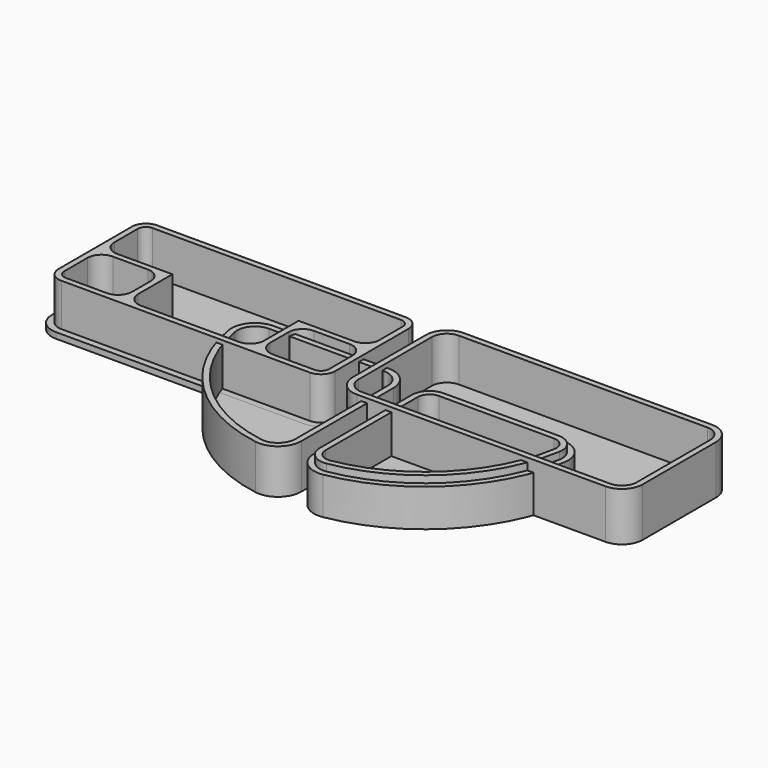
from build123d import *

# Parameters (mm, degrees)
F2_DEPTH = 3.175
F3_DEPTH = 24.13
F4_DEPTH = 20.32
F5_DEPTH = 24.13
F6_DEPTH = 3.175
F7_DEPTH = 26.275
F8_DEPTH = 26.5
F9_DEPTH = 3.175


# Not quite as in the source:
# - a feature names something its author has since deleted; it is built from what else it names


with BuildPart() as f2:
    # F1 (on Top) → F2 (new body)
    with BuildSketch(Plane.XY):
        with BuildLine():
            ThreePointArc((44.45, 31.75), (40.7302561211, 40.7302561211), (31.75, 44.45))
            Line((31.75, 44.45), (-30.6842132454, 44.45))
            ThreePointArc((-30.6842132454, 44.45), (-40.3839984664, 39.9478147495), (-43.2065821196, 29.6333333333))
            ThreePointArc((-43.2065821196, 29.6333333333), (-18.4117928475, -18.4117928475), (29.6333333333, -43.2065821196))
            ThreePointArc((29.6333333333, -43.2065821196), (39.9478147495, -40.3839984664), (44.45, -30.6842132454))
            Line((44.45, -30.6842132454), (44.45, 31.75))
        make_face()
        with BuildLine():
            ThreePointArc((31.75, 41.275), (38.4851920908, 38.4851920908), (41.275, 31.75))
            Line((41.275, 31.75), (41.275, -30.6842132454))
            ThreePointArc((41.275, -30.6842132454), (37.8983610621, -37.9590521611), (30.1625, -40.075989901))
            ThreePointArc((30.1625, -40.075989901), (-16.1667288172, -16.1667288172), (-40.075989901, 30.1625))
            ThreePointArc((-40.075989901, 30.1625), (-37.9590521611, 37.8983610621), (-30.6842132454, 41.275))
            Line((-30.6842132454, 41.275), (31.75, 41.275))
        make_face(mode=Mode.SUBTRACT)
        with BuildLine():
            Line((41.275, -30.6842132454), (41.275, 31.75))
            ThreePointArc((41.275, 31.75), (38.4851920908, 38.4851920908), (31.75, 41.275))
            Line((31.75, 41.275), (-30.6842132454, 41.275))
            ThreePointArc((-30.6842132454, 41.275), (-37.9590521611, 37.8983610621), (-40.075989901, 30.1625))
            ThreePointArc((-40.075989901, 30.1625), (-16.1667288172, -16.1667288172), (30.1625, -40.075989901))
            ThreePointArc((30.1625, -40.075989901), (37.8983610621, -37.9590521611), (41.275, -30.6842132454))
        make_face()
        with BuildLine():
            Line((-30.6842132454, 38.1), (31.75, 38.1))
            ThreePointArc((31.75, 38.1), (36.2401280605, 36.2401280605), (38.1, 31.75))
            Line((38.1, 31.75), (38.1, -30.6842132454))
            ThreePointArc((38.1, -30.6842132454), (35.8489073747, -35.5341058559), (30.6916666667, -36.9453976825))
            ThreePointArc((30.6916666667, -36.9453976825), (-13.9216647869, -13.9216647869), (-36.9453976825, 30.6916666667))
            ThreePointArc((-36.9453976825, 30.6916666667), (-35.5341058559, 35.8489073747), (-30.6842132454, 38.1))
        make_face(mode=Mode.SUBTRACT)
        with BuildLine():
            ThreePointArc((38.1, 31.75), (36.2401280605, 36.2401280605), (31.75, 38.1))
            Line((31.75, 38.1), (-30.6842132454, 38.1))
            ThreePointArc((-30.6842132454, 38.1), (-35.5341058559, 35.8489073747), (-36.9453976825, 30.6916666667))
            ThreePointArc((-36.9453976825, 30.6916666667), (-13.9216647869, -13.9216647869), (30.6916666667, -36.9453976825))
            ThreePointArc((30.6916666667, -36.9453976825), (35.8489073747, -35.5341058559), (38.1, -30.6842132454))
            Line((38.1, -30.6842132454), (38.1, 31.75))
        make_face()
    extrude(amount=F2_DEPTH)

    # F1 (on Top) → F3 (join)
    with BuildSketch(Plane.XY):
        with BuildLine():
            ThreePointArc((44.45, 31.75), (40.7302561211, 40.7302561211), (31.75, 44.45))
            Line((31.75, 44.45), (-30.6842132454, 44.45))
            ThreePointArc((-30.6842132454, 44.45), (-40.3839984664, 39.9478147495), (-43.2065821196, 29.6333333333))
            ThreePointArc((-43.2065821196, 29.6333333333), (-18.4117928475, -18.4117928475), (29.6333333333, -43.2065821196))
            ThreePointArc((29.6333333333, -43.2065821196), (39.9478147495, -40.3839984664), (44.45, -30.6842132454))
            Line((44.45, -30.6842132454), (44.45, 31.75))
        make_face()
        with BuildLine():
            ThreePointArc((31.75, 41.275), (38.4851920908, 38.4851920908), (41.275, 31.75))
            Line((41.275, 31.75), (41.275, -30.6842132454))
            ThreePointArc((41.275, -30.6842132454), (37.8983610621, -37.9590521611), (30.1625, -40.075989901))
            ThreePointArc((30.1625, -40.075989901), (-16.1667288172, -16.1667288172), (-40.075989901, 30.1625))
            ThreePointArc((-40.075989901, 30.1625), (-37.9590521611, 37.8983610621), (-30.6842132454, 41.275))
            Line((-30.6842132454, 41.275), (31.75, 41.275))
        make_face(mode=Mode.SUBTRACT)
    extrude(amount=F3_DEPTH)


with BuildPart() as f2b:
    # F1 (on Top) → F2, piece 2 (new body)
    with BuildSketch(Plane.XY):
        with BuildLine():
            Line((51.308, 31.75), (51.308, -30.6842132454))
            ThreePointArc((51.308, -30.6842132454), (55.8101852505, -40.3839984664), (66.1246666667, -43.2065821196))
            ThreePointArc((66.1246666667, -43.2065821196), (114.1697928475, -18.4117928475), (138.9645821196, 29.6333333333))
            ThreePointArc((138.9645821196, 29.6333333333), (136.1419984664, 39.9478147495), (126.4422132454, 44.45))
            Line((126.4422132454, 44.45), (64.008, 44.45))
            ThreePointArc((64.008, 44.45), (55.0277438789, 40.7302561211), (51.308, 31.75))
        make_face()
        with BuildLine():
            ThreePointArc((65.5955, -40.075989901), (57.8596389379, -37.9590521611), (54.483, -30.6842132454))
            Line((54.483, -30.6842132454), (54.483, 31.75))
            ThreePointArc((54.483, 31.75), (57.2728079092, 38.4851920908), (64.008, 41.275))
            Line((64.008, 41.275), (126.4422132454, 41.275))
            ThreePointArc((126.4422132454, 41.275), (133.7170521611, 37.8983610621), (135.833989901, 30.1625))
            ThreePointArc((135.833989901, 30.1625), (111.9247288172, -16.1667288172), (65.5955, -40.075989901))
        make_face(mode=Mode.SUBTRACT)
        with BuildLine():
            Line((54.483, 31.75), (54.483, -30.6842132454))
            ThreePointArc((54.483, -30.6842132454), (57.8596389379, -37.9590521611), (65.5955, -40.075989901))
            ThreePointArc((65.5955, -40.075989901), (111.9247288172, -16.1667288172), (135.833989901, 30.1625))
            ThreePointArc((135.833989901, 30.1625), (133.7170521611, 37.8983610621), (126.4422132454, 41.275))
            Line((126.4422132454, 41.275), (64.008, 41.275))
            ThreePointArc((64.008, 41.275), (57.2728079092, 38.4851920908), (54.483, 31.75))
        make_face()
        with BuildLine():
            ThreePointArc((65.0663333333, -36.9453976825), (59.9090926253, -35.5341058559), (57.658, -30.6842132454))
            Line((57.658, -30.6842132454), (57.658, 31.75))
            ThreePointArc((57.658, 31.75), (59.5178719395, 36.2401280605), (64.008, 38.1))
            Line((64.008, 38.1), (126.4422132454, 38.1))
            ThreePointArc((126.4422132454, 38.1), (131.2921058559, 35.8489073747), (132.7033976825, 30.6916666667))
            ThreePointArc((132.7033976825, 30.6916666667), (109.6796647869, -13.9216647869), (65.0663333333, -36.9453976825))
        make_face(mode=Mode.SUBTRACT)
        with BuildLine():
            Line((57.658, 31.75), (57.658, -30.6842132454))
            ThreePointArc((57.658, -30.6842132454), (59.9090926253, -35.5341058559), (65.0663333333, -36.9453976825))
            ThreePointArc((65.0663333333, -36.9453976825), (109.6796647869, -13.9216647869), (132.7033976825, 30.6916666667))
            ThreePointArc((132.7033976825, 30.6916666667), (131.2921058559, 35.8489073747), (126.4422132454, 38.1))
            Line((126.4422132454, 38.1), (64.008, 38.1))
            ThreePointArc((64.008, 38.1), (59.5178719395, 36.2401280605), (57.658, 31.75))
        make_face()
    extrude(amount=F2_DEPTH)

    # F1 (on Top) → F4 (join)
    with BuildSketch(Plane.XY):
        with BuildLine():
            Line((51.308, 31.75), (51.308, -30.6842132454))
            ThreePointArc((51.308, -30.6842132454), (55.8101852505, -40.3839984664), (66.1246666667, -43.2065821196))
            ThreePointArc((66.1246666667, -43.2065821196), (114.1697928475, -18.4117928475), (138.9645821196, 29.6333333333))
            ThreePointArc((138.9645821196, 29.6333333333), (136.1419984664, 39.9478147495), (126.4422132454, 44.45))
            Line((126.4422132454, 44.45), (64.008, 44.45))
            ThreePointArc((64.008, 44.45), (55.0277438789, 40.7302561211), (51.308, 31.75))
        make_face()
        with BuildLine():
            ThreePointArc((65.5955, -40.075989901), (57.8596389379, -37.9590521611), (54.483, -30.6842132454))
            Line((54.483, -30.6842132454), (54.483, 31.75))
            ThreePointArc((54.483, 31.75), (57.2728079092, 38.4851920908), (64.008, 41.275))
            Line((64.008, 41.275), (126.4422132454, 41.275))
            ThreePointArc((126.4422132454, 41.275), (133.7170521611, 37.8983610621), (135.833989901, 30.1625))
            ThreePointArc((135.833989901, 30.1625), (111.9247288172, -16.1667288172), (65.5955, -40.075989901))
        make_face(mode=Mode.SUBTRACT)
        with BuildLine():
            Line((54.483, 31.75), (54.483, -30.6842132454))
            ThreePointArc((54.483, -30.6842132454), (57.8596389379, -37.9590521611), (65.5955, -40.075989901))
            ThreePointArc((65.5955, -40.075989901), (111.9247288172, -16.1667288172), (135.833989901, 30.1625))
            ThreePointArc((135.833989901, 30.1625), (133.7170521611, 37.8983610621), (126.4422132454, 41.275))
            Line((126.4422132454, 41.275), (64.008, 41.275))
            ThreePointArc((64.008, 41.275), (57.2728079092, 38.4851920908), (54.483, 31.75))
        make_face()
        with BuildLine():
            ThreePointArc((65.0663333333, -36.9453976825), (59.9090926253, -35.5341058559), (57.658, -30.6842132454))
            Line((57.658, -30.6842132454), (57.658, 31.75))
            ThreePointArc((57.658, 31.75), (59.5178719395, 36.2401280605), (64.008, 38.1))
            Line((64.008, 38.1), (126.4422132454, 38.1))
            ThreePointArc((126.4422132454, 38.1), (131.2921058559, 35.8489073747), (132.7033976825, 30.6916666667))
            ThreePointArc((132.7033976825, 30.6916666667), (109.6796647869, -13.9216647869), (65.0663333333, -36.9453976825))
        make_face(mode=Mode.SUBTRACT)
    extrude(amount=F4_DEPTH)

    # F1 (on Top) → F5 (join)
    with BuildSketch(Plane.XY):
        with BuildLine():
            Line((54.483, 31.75), (54.483, -30.6842132454))
            ThreePointArc((54.483, -30.6842132454), (57.8596389379, -37.9590521611), (65.5955, -40.075989901))
            ThreePointArc((65.5955, -40.075989901), (111.9247288172, -16.1667288172), (135.833989901, 30.1625))
            ThreePointArc((135.833989901, 30.1625), (133.7170521611, 37.8983610621), (126.4422132454, 41.275))
            Line((126.4422132454, 41.275), (64.008, 41.275))
            ThreePointArc((64.008, 41.275), (57.2728079092, 38.4851920908), (54.483, 31.75))
        make_face()
        with BuildLine():
            ThreePointArc((65.0663333333, -36.9453976825), (59.9090926253, -35.5341058559), (57.658, -30.6842132454))
            Line((57.658, -30.6842132454), (57.658, 31.75))
            ThreePointArc((57.658, 31.75), (59.5178719395, 36.2401280605), (64.008, 38.1))
            Line((64.008, 38.1), (126.4422132454, 38.1))
            ThreePointArc((126.4422132454, 38.1), (131.2921058559, 35.8489073747), (132.7033976825, 30.6916666667))
            ThreePointArc((132.7033976825, 30.6916666667), (109.6796647869, -13.9216647869), (65.0663333333, -36.9453976825))
        make_face(mode=Mode.SUBTRACT)
    extrude(amount=F5_DEPTH)


with BuildPart() as f6:
    # F0 (on Top) → F6 (new body)
    with BuildSketch(Plane.XY):
        with BuildLine():
            ThreePointArc((38.9196167796, 86.1589387059), (30.9497646786, 82.8577178756), (27.6485438483, 74.8878657746))
            Line((27.6485438483, 74.8878657746), (27.6485438483, 25.1278657746))
            ThreePointArc((27.6485438483, 25.1278657746), (30.9497646786, 17.1580136737), (38.9196167796, 13.8567928433))
            Line((38.9196167796, 13.8567928433), (173.6796167796, 13.8567928433))
            ThreePointArc((173.6796167796, 13.8567928433), (181.6494688805, 17.1580136737), (184.9506897109, 25.1278657746))
            Line((184.9506897109, 25.1278657746), (184.9506897109, 74.8878657746))
            ThreePointArc((184.9506897109, 74.8878657746), (181.6494688805, 82.8577178756), (173.6796167796, 86.1589387059))
            Line((173.6796167796, 86.1589387059), (38.9196167796, 86.1589387059))
        make_face()
        with BuildLine():
            Line((30.7996167796, 25.1278657746), (30.7996167796, 74.8878657746))
            ThreePointArc((30.7996167796, 74.8878657746), (33.1779097163, 80.6295728379), (38.9196167796, 83.0078657746))
            Line((38.9196167796, 83.0078657746), (173.6796167796, 83.0078657746))
            ThreePointArc((173.6796167796, 83.0078657746), (179.4213238428, 80.6295728379), (181.7996167796, 74.8878657746))
            Line((181.7996167796, 74.8878657746), (181.7996167796, 25.1278657746))
            ThreePointArc((181.7996167796, 25.1278657746), (179.4213238428, 19.3861587114), (173.6796167796, 17.0078657746))
            Line((173.6796167796, 17.0078657746), (38.9196167796, 17.0078657746))
            ThreePointArc((38.9196167796, 17.0078657746), (33.1779097163, 19.3861587114), (30.7996167796, 25.1278657746))
        make_face(mode=Mode.SUBTRACT)
        with BuildLine():
            ThreePointArc((38.9196167796, 83.0078657746), (33.1779097163, 80.6295728379), (30.7996167796, 74.8878657746))
            Line((30.7996167796, 74.8878657746), (30.7996167796, 25.1278657746))
            ThreePointArc((30.7996167796, 25.1278657746), (33.1779097163, 19.3861587114), (38.9196167796, 17.0078657746))
            Line((38.9196167796, 17.0078657746), (173.6796167796, 17.0078657746))
            ThreePointArc((173.6796167796, 17.0078657746), (179.4213238428, 19.3861587114), (181.7996167796, 25.1278657746))
            Line((181.7996167796, 25.1278657746), (181.7996167796, 74.8878657746))
            ThreePointArc((181.7996167796, 74.8878657746), (179.4213238428, 80.6295728379), (173.6796167796, 83.0078657746))
            Line((173.6796167796, 83.0078657746), (38.9196167796, 83.0078657746))
        make_face()
    extrude(amount=F6_DEPTH)

    # F0 (on Top) → F8 (join)
    with BuildSketch(Plane.XY):
        with BuildLine():
            ThreePointArc((38.9196167796, 86.1589387059), (30.9497646786, 82.8577178756), (27.6485438483, 74.8878657746))
            Line((27.6485438483, 74.8878657746), (27.6485438483, 25.1278657746))
            ThreePointArc((27.6485438483, 25.1278657746), (30.9497646786, 17.1580136737), (38.9196167796, 13.8567928433))
            Line((38.9196167796, 13.8567928433), (173.6796167796, 13.8567928433))
            ThreePointArc((173.6796167796, 13.8567928433), (181.6494688805, 17.1580136737), (184.9506897109, 25.1278657746))
            Line((184.9506897109, 25.1278657746), (184.9506897109, 74.8878657746))
            ThreePointArc((184.9506897109, 74.8878657746), (181.6494688805, 82.8577178756), (173.6796167796, 86.1589387059))
            Line((173.6796167796, 86.1589387059), (38.9196167796, 86.1589387059))
        make_face()
        with BuildLine():
            Line((30.7996167796, 25.1278657746), (30.7996167796, 74.8878657746))
            ThreePointArc((30.7996167796, 74.8878657746), (33.1779097163, 80.6295728379), (38.9196167796, 83.0078657746))
            Line((38.9196167796, 83.0078657746), (173.6796167796, 83.0078657746))
            ThreePointArc((173.6796167796, 83.0078657746), (179.4213238428, 80.6295728379), (181.7996167796, 74.8878657746))
            Line((181.7996167796, 74.8878657746), (181.7996167796, 25.1278657746))
            ThreePointArc((181.7996167796, 25.1278657746), (179.4213238428, 19.3861587114), (173.6796167796, 17.0078657746))
            Line((173.6796167796, 17.0078657746), (38.9196167796, 17.0078657746))
            ThreePointArc((38.9196167796, 17.0078657746), (33.1779097163, 19.3861587114), (30.7996167796, 25.1278657746))
        make_face(mode=Mode.SUBTRACT)
    extrude(amount=F8_DEPTH)


with BuildPart() as f6b:
    # F0 (on Top) → F6, piece 2 (new body)
    with BuildSketch(Plane.XY):
        with BuildLine():
            Line((-124.2883832204, 17.5078657746), (10.4716167796, 17.5078657746))
            ThreePointArc((10.4716167796, 17.5078657746), (15.8597704522, 19.739712102), (18.0916167796, 25.1278657746))
            Line((18.0916167796, 25.1278657746), (18.0916167796, 74.8878657746))
            ThreePointArc((18.0916167796, 74.8878657746), (15.8597704522, 80.2760194473), (10.4716167796, 82.5078657746))
            Line((10.4716167796, 82.5078657746), (-124.2883832204, 82.5078657746))
            ThreePointArc((-124.2883832204, 82.5078657746), (-129.6765368931, 80.2760194473), (-131.9083832204, 74.8878657746))
            Line((-131.9083832204, 74.8878657746), (-131.9083832204, 25.1278657746))
            ThreePointArc((-131.9083832204, 25.1278657746), (-129.6765368931, 19.739712102), (-124.2883832204, 17.5078657746))
        make_face()
        with BuildLine():
            Line((-128.7333832204, 25.1278657746), (-128.7333832204, 40.8003657746))
            ThreePointArc((-128.7333832204, 40.8003657746), (-126.5015368931, 46.1885194473), (-121.1133832204, 48.4203657746))
            Line((-121.1133832204, 48.4203657746), (-102.1007441217, 48.4203657746))
            ThreePointArc((-102.1007441217, 48.4203657746), (-96.708055914, 46.1839810928), (-94.4807549245, 40.7875347756))
            Line((-94.4807549245, 40.7875347756), (-94.5017989715, 28.2900347756))
            ThreePointArc((-94.5017989715, 28.2900347756), (-96.7381728506, 22.9101775668), (-102.1217881687, 20.6828657746))
            Line((-102.1217881687, 20.6828657746), (-124.2883832204, 20.6828657746))
            ThreePointArc((-124.2883832204, 20.6828657746), (-127.4314728628, 21.9847761323), (-128.7333832204, 25.1278657746))
        make_face(mode=Mode.SUBTRACT)
        with BuildLine():
            ThreePointArc((10.4716167796, 79.3328657746), (13.6147064219, 78.030955417), (14.9166167796, 74.8878657746))
            Line((14.9166167796, 74.8878657746), (14.9166167796, 59.2153657746))
            ThreePointArc((14.9166167796, 59.2153657746), (12.6847704522, 53.827212102), (7.2966167796, 51.5953657746))
            Line((7.2966167796, 51.5953657746), (-22.8660074278, 51.5718185735))
            Line((-22.8660074278, 51.5718185735), (-22.8478419423, 28.3028657746))
            ThreePointArc((-22.8478419423, 28.3028657746), (-25.0796882697, 22.914712102), (-30.4678419423, 20.6828657746))
            Line((-30.4678419423, 20.6828657746), (-83.6065935341, 20.6828657746))
            ThreePointArc((-83.6065935341, 20.6828657746), (-88.9992817419, 22.9192504565), (-91.2265827313, 28.3156967737))
            Line((-91.2265827313, 28.3156967737), (-91.2446965263, 51.518437053))
            Line((-91.2446965263, 51.518437053), (-121.0133833622, 51.4951973888))
            ThreePointArc((-121.0133833622, 51.4951973888), (-126.4660648418, 53.6911474728), (-128.7333832204, 59.1145411944))
            Line((-128.7333832204, 59.1145411944), (-128.7333832204, 74.8878657746))
            ThreePointArc((-128.7333832204, 74.8878657746), (-127.4314728628, 78.030955417), (-124.2883832204, 79.3328657746))
            Line((-124.2883832204, 79.3328657746), (10.4716167796, 79.3328657746))
        make_face(mode=Mode.SUBTRACT)
        with BuildLine():
            ThreePointArc((7.2966167796, 48.4203657746), (12.6847704522, 46.1885194473), (14.9166167796, 40.8003657746))
            Line((14.9166167796, 40.8003657746), (14.9166167796, 25.1278657746))
            ThreePointArc((14.9166167796, 25.1278657746), (13.6147064219, 21.9847761323), (10.4716167796, 20.6828657746))
            Line((10.4716167796, 20.6828657746), (-12.0528419423, 20.6828657746))
            ThreePointArc((-12.0528419423, 20.6828657746), (-17.440995615, 22.914712102), (-19.6728419423, 28.3028657746))
            Line((-19.6728419423, 28.3028657746), (-19.6728419423, 40.8003657746))
            ThreePointArc((-19.6728419423, 40.8003657746), (-17.440995615, 46.1885194473), (-12.0528419423, 48.4203657746))
            Line((-12.0528419423, 48.4203657746), (7.2966167796, 48.4203657746))
        make_face(mode=Mode.SUBTRACT)
        with BuildLine():
            Line((14.9166167796, 25.1278657746), (14.9166167796, 40.8003657746))
            ThreePointArc((14.9166167796, 40.8003657746), (12.6847704522, 46.1885194473), (7.2966167796, 48.4203657746))
            Line((7.2966167796, 48.4203657746), (-12.0528419423, 48.4203657746))
            ThreePointArc((-12.0528419423, 48.4203657746), (-17.440995615, 46.1885194473), (-19.6728419423, 40.8003657746))
            Line((-19.6728419423, 40.8003657746), (-19.6728419423, 28.3028657746))
            ThreePointArc((-19.6728419423, 28.3028657746), (-17.440995615, 22.914712102), (-12.0528419423, 20.6828657746))
            Line((-12.0528419423, 20.6828657746), (10.4716167796, 20.6828657746))
            ThreePointArc((10.4716167796, 20.6828657746), (13.6147064219, 21.9847761323), (14.9166167796, 25.1278657746))
        make_face()
        with BuildLine():
            Line((14.9166167796, 59.2153657746), (14.9166167796, 74.8878657746))
            ThreePointArc((14.9166167796, 74.8878657746), (13.6147064219, 78.030955417), (10.4716167796, 79.3328657746))
            Line((10.4716167796, 79.3328657746), (-124.2883832204, 79.3328657746))
            ThreePointArc((-124.2883832204, 79.3328657746), (-127.4314728628, 78.030955417), (-128.7333832204, 74.8878657746))
            Line((-128.7333832204, 74.8878657746), (-128.7333832204, 59.1145411944))
            ThreePointArc((-128.7333832204, 59.1145411944), (-126.4660648418, 53.6911474728), (-121.0133833622, 51.4951973888))
            Line((-121.0133833622, 51.4951973888), (-91.2446965263, 51.518437053))
            Line((-91.2446965263, 51.518437053), (-22.8660074278, 51.5718185735))
            Line((-22.8660074278, 51.5718185735), (7.2966167796, 51.5953657746))
            ThreePointArc((7.2966167796, 51.5953657746), (12.6847704522, 53.827212102), (14.9166167796, 59.2153657746))
        make_face()
        with BuildLine():
            ThreePointArc((-121.1133832204, 48.4203657746), (-126.5015368931, 46.1885194473), (-128.7333832204, 40.8003657746))
            Line((-128.7333832204, 40.8003657746), (-128.7333832204, 25.1278657746))
            ThreePointArc((-128.7333832204, 25.1278657746), (-127.4314728628, 21.9847761323), (-124.2883832204, 20.6828657746))
            Line((-124.2883832204, 20.6828657746), (-102.1217881687, 20.6828657746))
            ThreePointArc((-102.1217881687, 20.6828657746), (-96.7381728506, 22.9101775668), (-94.5017989715, 28.2900347756))
            Line((-94.5017989715, 28.2900347756), (-94.4807549245, 40.7875347756))
            ThreePointArc((-94.4807549245, 40.7875347756), (-96.708055914, 46.1839810928), (-102.1007441217, 48.4203657746))
            Line((-102.1007441217, 48.4203657746), (-121.1133832204, 48.4203657746))
        make_face()
        with BuildLine():
            Line((-22.8478419423, 28.3028657746), (-22.8660074278, 51.5718185735))
            Line((-22.8660074278, 51.5718185735), (-91.2446965263, 51.518437053))
            Line((-91.2446965263, 51.518437053), (-91.2265827313, 28.3156967737))
            ThreePointArc((-91.2265827313, 28.3156967737), (-88.9992817419, 22.9192504565), (-83.6065935341, 20.6828657746))
            Line((-83.6065935341, 20.6828657746), (-30.4678419423, 20.6828657746))
            ThreePointArc((-30.4678419423, 20.6828657746), (-25.0796882697, 22.914712102), (-22.8478419423, 28.3028657746))
        make_face()
    extrude(amount=F6_DEPTH)

    # F0 (on Top) → F7 (join)
    with BuildSketch(Plane.XY):
        with BuildLine():
            Line((-124.2883832204, 17.5078657746), (10.4716167796, 17.5078657746))
            ThreePointArc((10.4716167796, 17.5078657746), (15.8597704522, 19.739712102), (18.0916167796, 25.1278657746))
            Line((18.0916167796, 25.1278657746), (18.0916167796, 74.8878657746))
            ThreePointArc((18.0916167796, 74.8878657746), (15.8597704522, 80.2760194473), (10.4716167796, 82.5078657746))
            Line((10.4716167796, 82.5078657746), (-124.2883832204, 82.5078657746))
            ThreePointArc((-124.2883832204, 82.5078657746), (-129.6765368931, 80.2760194473), (-131.9083832204, 74.8878657746))
            Line((-131.9083832204, 74.8878657746), (-131.9083832204, 25.1278657746))
            ThreePointArc((-131.9083832204, 25.1278657746), (-129.6765368931, 19.739712102), (-124.2883832204, 17.5078657746))
        make_face()
        with BuildLine():
            Line((-128.7333832204, 25.1278657746), (-128.7333832204, 40.8003657746))
            ThreePointArc((-128.7333832204, 40.8003657746), (-126.5015368931, 46.1885194473), (-121.1133832204, 48.4203657746))
            Line((-121.1133832204, 48.4203657746), (-102.1007441217, 48.4203657746))
            ThreePointArc((-102.1007441217, 48.4203657746), (-96.708055914, 46.1839810928), (-94.4807549245, 40.7875347756))
            Line((-94.4807549245, 40.7875347756), (-94.5017989715, 28.2900347756))
            ThreePointArc((-94.5017989715, 28.2900347756), (-96.7381728506, 22.9101775668), (-102.1217881687, 20.6828657746))
            Line((-102.1217881687, 20.6828657746), (-124.2883832204, 20.6828657746))
            ThreePointArc((-124.2883832204, 20.6828657746), (-127.4314728628, 21.9847761323), (-128.7333832204, 25.1278657746))
        make_face(mode=Mode.SUBTRACT)
        with BuildLine():
            ThreePointArc((10.4716167796, 79.3328657746), (13.6147064219, 78.030955417), (14.9166167796, 74.8878657746))
            Line((14.9166167796, 74.8878657746), (14.9166167796, 59.2153657746))
            ThreePointArc((14.9166167796, 59.2153657746), (12.6847704522, 53.827212102), (7.2966167796, 51.5953657746))
            Line((7.2966167796, 51.5953657746), (-22.8660074278, 51.5718185735))
            Line((-22.8660074278, 51.5718185735), (-22.8478419423, 28.3028657746))
            ThreePointArc((-22.8478419423, 28.3028657746), (-25.0796882697, 22.914712102), (-30.4678419423, 20.6828657746))
            Line((-30.4678419423, 20.6828657746), (-83.6065935341, 20.6828657746))
            ThreePointArc((-83.6065935341, 20.6828657746), (-88.9992817419, 22.9192504565), (-91.2265827313, 28.3156967737))
            Line((-91.2265827313, 28.3156967737), (-91.2446965263, 51.518437053))
            Line((-91.2446965263, 51.518437053), (-121.0133833622, 51.4951973888))
            ThreePointArc((-121.0133833622, 51.4951973888), (-126.4660648418, 53.6911474728), (-128.7333832204, 59.1145411944))
            Line((-128.7333832204, 59.1145411944), (-128.7333832204, 74.8878657746))
            ThreePointArc((-128.7333832204, 74.8878657746), (-127.4314728628, 78.030955417), (-124.2883832204, 79.3328657746))
            Line((-124.2883832204, 79.3328657746), (10.4716167796, 79.3328657746))
        make_face(mode=Mode.SUBTRACT)
        with BuildLine():
            ThreePointArc((7.2966167796, 48.4203657746), (12.6847704522, 46.1885194473), (14.9166167796, 40.8003657746))
            Line((14.9166167796, 40.8003657746), (14.9166167796, 25.1278657746))
            ThreePointArc((14.9166167796, 25.1278657746), (13.6147064219, 21.9847761323), (10.4716167796, 20.6828657746))
            Line((10.4716167796, 20.6828657746), (-12.0528419423, 20.6828657746))
            ThreePointArc((-12.0528419423, 20.6828657746), (-17.440995615, 22.914712102), (-19.6728419423, 28.3028657746))
            Line((-19.6728419423, 28.3028657746), (-19.6728419423, 40.8003657746))
            ThreePointArc((-19.6728419423, 40.8003657746), (-17.440995615, 46.1885194473), (-12.0528419423, 48.4203657746))
            Line((-12.0528419423, 48.4203657746), (7.2966167796, 48.4203657746))
        make_face(mode=Mode.SUBTRACT)
    extrude(amount=F7_DEPTH)

    # F0 (on Top) → F9 (join)
    with BuildSketch(Plane.XY):
        with BuildLine():
            Line((21.6916159809, 25.1278657746), (21.6916159809, 74.8878657746))
            ThreePointArc((21.6916159809, 74.8878657746), (18.4053542997, 82.8216032948), (10.4716167796, 86.1078649759))
            Line((10.4716167796, 86.1078649759), (-124.2883832204, 86.1078649759))
            ThreePointArc((-124.2883832204, 86.1078649759), (-132.2221207406, 82.8216032948), (-135.5083824217, 74.8878657746))
            Line((-135.5083824217, 74.8878657746), (-135.5083824217, 25.1278657746))
            ThreePointArc((-135.5083824217, 25.1278657746), (-132.2221207406, 17.1941282545), (-124.2883832204, 13.9078665733))
            Line((-124.2883832204, 13.9078665733), (10.4716167796, 13.9078665733))
            ThreePointArc((10.4716167796, 13.9078665733), (18.4053542997, 17.1941282545), (21.6916159809, 25.1278657746))
        make_face()
        with BuildLine():
            ThreePointArc((18.0916167796, 25.1278657746), (15.8597704522, 19.739712102), (10.4716167796, 17.5078657746))
            Line((10.4716167796, 17.5078657746), (-124.2883832204, 17.5078657746))
            ThreePointArc((-124.2883832204, 17.5078657746), (-129.6765368931, 19.739712102), (-131.9083832204, 25.1278657746))
            Line((-131.9083832204, 25.1278657746), (-131.9083832204, 74.8878657746))
            ThreePointArc((-131.9083832204, 74.8878657746), (-129.6765368931, 80.2760194473), (-124.2883832204, 82.5078657746))
            Line((-124.2883832204, 82.5078657746), (10.4716167796, 82.5078657746))
            ThreePointArc((10.4716167796, 82.5078657746), (15.8597704522, 80.2760194473), (18.0916167796, 74.8878657746))
            Line((18.0916167796, 74.8878657746), (18.0916167796, 25.1278657746))
        make_face(mode=Mode.SUBTRACT)
    extrude(amount=F9_DEPTH)


solid = Compound([f2.part, f2b.part, f6.part, f6b.part])
